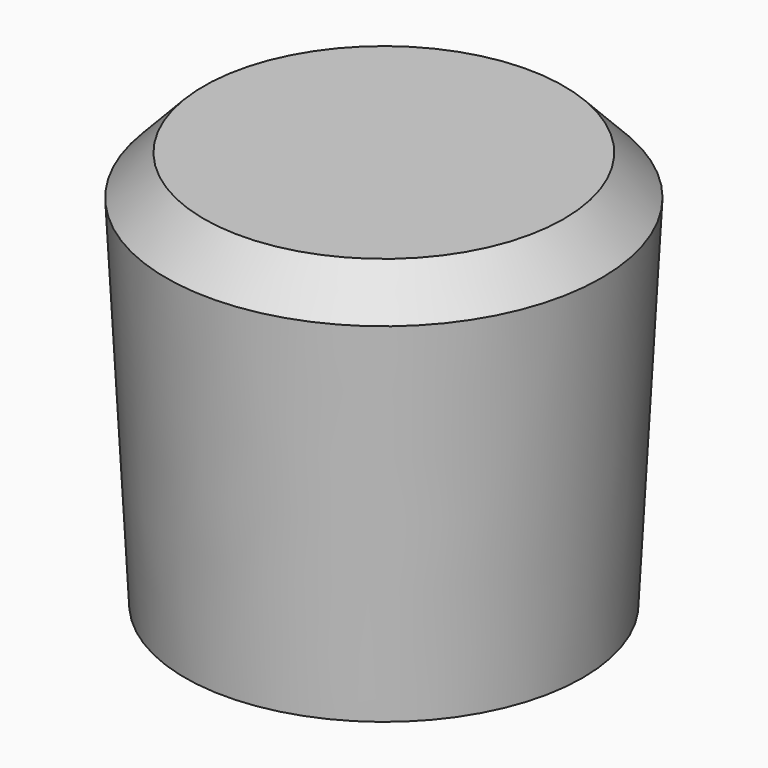
from build123d import *

# Parameters (mm, degrees)
F0_R     = 25.4
F1_DEPTH = 50.8
F1_TAPER = -3


# Not quite as in the source:
# - a fillet or chamfer that OpenCascade refuses, or shapes differently, is made with other operations: its cross-section is extruded or revolved along the edge and cut away or added


with BuildPart() as f1:
    # F0 (on Top) → F1 (new body)
    with BuildSketch(Plane.XY):
        Circle(F0_R)
    extrude(amount=F1_DEPTH, taper=F1_TAPER)

    # F2: chamfer of 5.08 on 1 edges, made by hand

    # F2_s1 → F2_t2 (revolve, cut)
    with BuildSketch(Plane.XZ):
        Polygon((27.7964485299, 45.7269619634), (22.9823151876, 50.8), (28.0623151876, 50.8), align=None)
    revolve(axis=Axis((0, 0, 50.8), (0, 0, -1)), mode=Mode.SUBTRACT)


solid = f1.part
